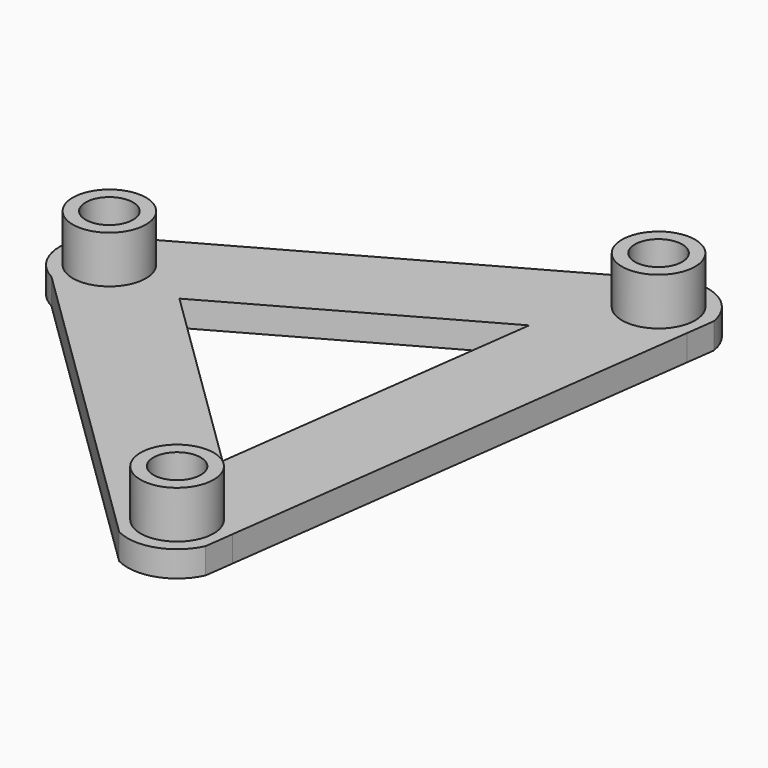
from build123d import *

# Parameters (mm, degrees)
F0_R     = 4.25
F0_R_2   = 2.75
F1_DEPTH = 3
F2_DEPTH = 8.5


# Not quite as in the source:
# - a feature names something its author has since deleted; it is built from what else it names


with BuildPart() as f1:
    # F0 (on Top) → F1 (new body)
    with BuildSketch(Plane.XY):
        with BuildLine():
            ThreePointArc((-20.0475404255, -5.1050880284), (-14.4143064726, -4.9130538455), (-11.6516802209, 0))
            ThreePointArc((-11.6516802209, 0), (-13.7942703105, 4.4776214376), (-18.6252780431, 5.6183011996))
            ThreePointArc((-18.6252780431, 5.6183011996), (-23.1017631579, 0.7560122426), (-20.0475404255, -5.1050880284))
        make_face()
        with Locations((-17.4016802209, 0)):
            Circle(F0_R, mode=Mode.SUBTRACT)
        with BuildLine():
            ThreePointArc((-18.6252780431, 5.6183011996), (-13.7942703105, 4.4776214376), (-11.6516802209, 0))
            ThreePointArc((-11.6516802209, 0), (-14.4143064726, -4.9130538455), (-20.0475404255, -5.1050880284))
            Line((-20.0475404255, -5.1050880284), (13.6632948995, -38.0643911727))
            ThreePointArc((13.6632948995, -38.0643911727), (16.8311240547, -29.8688761508), (24.3801958358, -34.3647768698))
            Line((24.3801958358, -34.3647768698), (31.8937613277, 22.2850285764))
            ThreePointArc((31.8937613277, 22.2850285764), (23.4337103416, 19.9124465773), (22.5117964167, 28.6503915729))
            Line((22.5117964167, 28.6503915729), (-18.6252780431, 5.6183011996))
        make_face()
        Polygon((14.6992403306, -23.6933170767), (-8.2995714993, -1.2072290356), (19.7657026362, 14.5061375255), align=None, mode=Mode.SUBTRACT)
        with BuildLine():
            ThreePointArc((32.3347594316, 25.6100088156), (28.3621582746, 30.1635639823), (22.5117964167, 28.6503915729))
            ThreePointArc((22.5117964167, 28.6503915729), (23.4337103416, 19.9124465773), (31.8937613277, 22.2850285764))
            Line((31.8937613277, 22.2850285764), (32.3347594316, 25.6100088156))
        make_face()
        with Locations((26.6620065254, 24.670660922)):
            Circle(F0_R, mode=Mode.SUBTRACT)
        with BuildLine():
            ThreePointArc((24.3801958358, -34.3647768698), (16.8311240547, -29.8688761508), (13.6632948995, -38.0643911727))
            Line((13.6632948995, -38.0643911727), (16.0615827249, -40.4092127917))
            ThreePointArc((16.0615827249, -40.4092127917), (20.5837618045, -40.7393733758), (23.9391977319, -37.6897571089))
            Line((23.9391977319, -37.6897571089), (24.3801958358, -34.3647768698))
        make_face()
        with Locations((18.7074429296, -35.3041247633)):
            Circle(F0_R, mode=Mode.SUBTRACT)
        with Locations((-17.4016802209, 0)):
            Circle(F0_R)
        with Locations((-17.4016802209, 0)):
            Circle(F0_R_2, mode=Mode.SUBTRACT)
        with Locations((26.6620065254, 24.670660922)):
            Circle(F0_R)
        with Locations((26.6620065254, 24.670660922)):
            Circle(F0_R_2, mode=Mode.SUBTRACT)
        with Locations((18.7074429296, -35.3041247633)):
            Circle(F0_R)
        with Locations((18.7074429296, -35.3041247633)):
            Circle(F0_R_2, mode=Mode.SUBTRACT)
    extrude(amount=F1_DEPTH)

    # F0 (on Top) → F2 (join)
    with BuildSketch(Plane.XY):
        with Locations((26.6620065254, 24.670660922)):
            Circle(F0_R)
        with Locations((26.6620065254, 24.670660922)):
            Circle(F0_R_2, mode=Mode.SUBTRACT)
        with Locations((-17.4016802209, 0)):
            Circle(F0_R)
        with Locations((-17.4016802209, 0)):
            Circle(F0_R_2, mode=Mode.SUBTRACT)
        with Locations((18.7074429296, -35.3041247633)):
            Circle(F0_R)
        with Locations((18.7074429296, -35.3041247633)):
            Circle(F0_R_2, mode=Mode.SUBTRACT)
    extrude(amount=F2_DEPTH)


solid = f1.part
